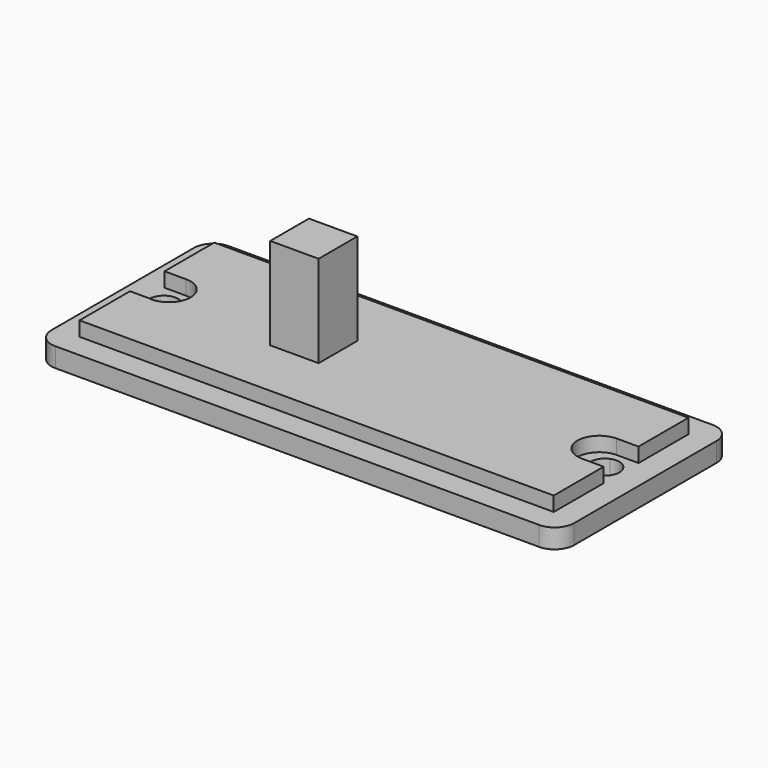
from build123d import *

# Parameters (mm, degrees)
F0_W     = 54
F0_H     = 22.4
F0_W_2   = 5
F0_H_2   = 5
F1_DEPTH = 2
F2_DEPTH = 13
F3_DEPTH = 3.5
F4_R     = 2


# Not quite as in the source:
# - a feature names something its author has since deleted; it is built from what else it names


with BuildPart() as f1:
    # F0 (on Top) → F1 (new body)
    with BuildSketch(Plane.XY):
        with Locations((1.3893617413, 0.829365923)):
            Rectangle(F0_W, F0_H)
        Polygon((-23.1106382587, 3.1091097071), (-23.1106382587, 9.529365923), (25.8893617413, 9.529365923), (25.8893617413, 3.079365923), (25.8893617413, 0.829365923), (25.8893617413, -1.420634077), (25.8893617413, -7.870634077), (-23.1106382587, -7.870634077), (-23.1106382587, -1.3557597995), (-23.1106382587, 0.859365923), align=None, mode=Mode.SUBTRACT)
        with BuildLine():
            Line((25.8893617413, 9.529365923), (-23.1106382587, 9.529365923))
            Line((-23.1106382587, 9.529365923), (-23.1106382587, 3.1091097071))
            Line((-23.1106382587, 3.1091097071), (-20.8945927259, 3.1091097071))
            ThreePointArc((-20.8945927259, 3.1091097071), (-19.2816983534, 2.4623159458), (-18.6106382587, 0.859365923))
            ThreePointArc((-18.6106382587, 0.859365923), (-19.4158848712, -0.8655073041), (-21.2552495026, -1.3557597995))
            Line((-21.2552495026, -1.3557597995), (-23.1106382587, -1.3557597995))
            Line((-23.1106382587, -1.3557597995), (-23.1106382587, -7.870634077))
            Line((-23.1106382587, -7.870634077), (25.8893617413, -7.870634077))
            Line((25.8893617413, -7.870634077), (25.8893617413, -1.420634077))
            Line((25.8893617413, -1.420634077), (23.6393617413, -1.420634077))
            ThreePointArc((23.6393617413, -1.420634077), (21.3893617413, 0.829365923), (23.6393617413, 3.079365923))
            Line((23.6393617413, 3.079365923), (25.8893617413, 3.079365923))
            Line((25.8893617413, 3.079365923), (25.8893617413, 9.529365923))
        make_face()
        with Locations((-5.8658428788, 0.829365923)):
            Rectangle(F0_W_2, F0_H_2, mode=Mode.SUBTRACT)
        with BuildLine():
            Line((-20.8945927259, 3.1091097071), (-23.1106382587, 3.1091097071))
            Line((-23.1106382587, 3.1091097071), (-23.1106382587, 0.859365923))
            ThreePointArc((-23.1106382587, 0.859365923), (-22.4635882815, 2.4383058282), (-20.8945927259, 3.1091097071))
        make_face()
        with BuildLine():
            Line((25.8893617413, 0.829365923), (25.8893617413, 3.079365923))
            Line((25.8893617413, 3.079365923), (23.6393617413, 3.079365923))
            ThreePointArc((23.6393617413, 3.079365923), (25.230351999, 2.4203561806), (25.8893617413, 0.829365923))
        make_face()
        with BuildLine():
            ThreePointArc((-21.2552495026, -1.3557597995), (-22.5855114857, -0.5853874645), (-23.1106382587, 0.859365923))
            Line((-23.1106382587, 0.859365923), (-23.1106382587, -1.3557597995))
            Line((-23.1106382587, -1.3557597995), (-21.2552495026, -1.3557597995))
        make_face()
        with BuildLine():
            ThreePointArc((-20.8945927259, 3.1091097071), (-22.4635882815, 2.4383058282), (-23.1106382587, 0.859365923))
            ThreePointArc((-23.1106382587, 0.859365923), (-22.5855114857, -0.5853874645), (-21.2552495026, -1.3557597995))
            Line((-21.2552495026, -1.3557597995), (-20.8945927259, -1.3557597995))
            Line((-20.8945927259, -1.3557597995), (-20.8945927259, -0.5963975782))
            ThreePointArc((-20.8945927259, -0.5963975782), (-22.8606382587, 0.829365923), (-20.8945927259, 2.2551294242))
            Line((-20.8945927259, 2.2551294242), (-20.8945927259, 3.1091097071))
        make_face()
        with BuildLine():
            ThreePointArc((-18.6106382587, 0.859365923), (-19.2816983534, 2.4623159458), (-20.8945927259, 3.1091097071))
            Line((-20.8945927259, 3.1091097071), (-20.8945927259, 2.2551294242))
            ThreePointArc((-20.8945927259, 2.2551294242), (-20.1463342813, 1.7099713115), (-19.8606382587, 0.829365923))
            ThreePointArc((-19.8606382587, 0.829365923), (-20.1463342813, -0.0512394656), (-20.8945927259, -0.5963975782))
            Line((-20.8945927259, -0.5963975782), (-20.8945927259, -1.3557597995))
            Line((-20.8945927259, -1.3557597995), (-21.2552495026, -1.3557597995))
            ThreePointArc((-21.2552495026, -1.3557597995), (-19.4158848712, -0.8655073041), (-18.6106382587, 0.859365923))
        make_face()
        with BuildLine():
            ThreePointArc((23.6393617413, -1.420634077), (25.230351999, -0.7616243347), (25.8893617413, 0.829365923))
            ThreePointArc((25.8893617413, 0.829365923), (25.230351999, 2.4203561806), (23.6393617413, 3.079365923))
            Line((23.6393617413, 3.079365923), (23.6393617413, 2.2174858052))
            ThreePointArc((23.6393617413, 2.2174858052), (25.043666155, 2.0748896863), (25.7078010014, 0.829365923))
            ThreePointArc((25.7078010014, 0.829365923), (25.043666155, -0.4161578404), (23.6393617413, -0.5587539593))
            Line((23.6393617413, -0.5587539593), (23.6393617413, -1.420634077))
        make_face()
        with BuildLine():
            Line((25.8893617413, -1.420634077), (25.8893617413, 0.829365923))
            ThreePointArc((25.8893617413, 0.829365923), (25.230351999, -0.7616243347), (23.6393617413, -1.420634077))
            Line((23.6393617413, -1.420634077), (25.8893617413, -1.420634077))
        make_face()
        with BuildLine():
            Line((23.6393617413, 2.2174858052), (23.6393617413, 3.079365923))
            ThreePointArc((23.6393617413, 3.079365923), (21.3893617413, 0.829365923), (23.6393617413, -1.420634077))
            Line((23.6393617413, -1.420634077), (23.6393617413, -0.5587539593))
            ThreePointArc((23.6393617413, -0.5587539593), (22.7078010014, 0.829365923), (23.6393617413, 2.2174858052))
        make_face()
        with Locations((-5.8658428788, 0.829365923)):
            Rectangle(F0_W_2, F0_H_2)
    extrude(amount=F1_DEPTH)

    # F0 (on Top) → F2 (join)
    with BuildSketch(Plane.XY):
        with Locations((-5.8658428788, 0.829365923)):
            Rectangle(F0_W_2, F0_H_2)
    extrude(amount=F2_DEPTH)

    # F0 (on Top) → F3 (join)
    with BuildSketch(Plane.XY):
        with BuildLine():
            Line((25.8893617413, 9.529365923), (-23.1106382587, 9.529365923))
            Line((-23.1106382587, 9.529365923), (-23.1106382587, 3.1091097071))
            Line((-23.1106382587, 3.1091097071), (-20.8945927259, 3.1091097071))
            ThreePointArc((-20.8945927259, 3.1091097071), (-19.2816983534, 2.4623159458), (-18.6106382587, 0.859365923))
            ThreePointArc((-18.6106382587, 0.859365923), (-19.4158848712, -0.8655073041), (-21.2552495026, -1.3557597995))
            Line((-21.2552495026, -1.3557597995), (-23.1106382587, -1.3557597995))
            Line((-23.1106382587, -1.3557597995), (-23.1106382587, -7.870634077))
            Line((-23.1106382587, -7.870634077), (25.8893617413, -7.870634077))
            Line((25.8893617413, -7.870634077), (25.8893617413, -1.420634077))
            Line((25.8893617413, -1.420634077), (23.6393617413, -1.420634077))
            ThreePointArc((23.6393617413, -1.420634077), (21.3893617413, 0.829365923), (23.6393617413, 3.079365923))
            Line((23.6393617413, 3.079365923), (25.8893617413, 3.079365923))
            Line((25.8893617413, 3.079365923), (25.8893617413, 9.529365923))
        make_face()
        with Locations((-5.8658428788, 0.829365923)):
            Rectangle(F0_W_2, F0_H_2, mode=Mode.SUBTRACT)
        with Locations((-5.8658428788, 0.829365923)):
            Rectangle(F0_W_2, F0_H_2)
    extrude(amount=F3_DEPTH)

    # F4
    f4_edges = [f1.edges().sort_by_distance(p)[0] for p in [
        (-25.610638, 12.029366, 1),
        (-25.610638, -10.370634, 1),
        (28.389362, 12.029366, 1),
        (28.389362, -10.370634, 1),
    ]]
    fillet(f4_edges, radius=F4_R)


solid = f1.part
